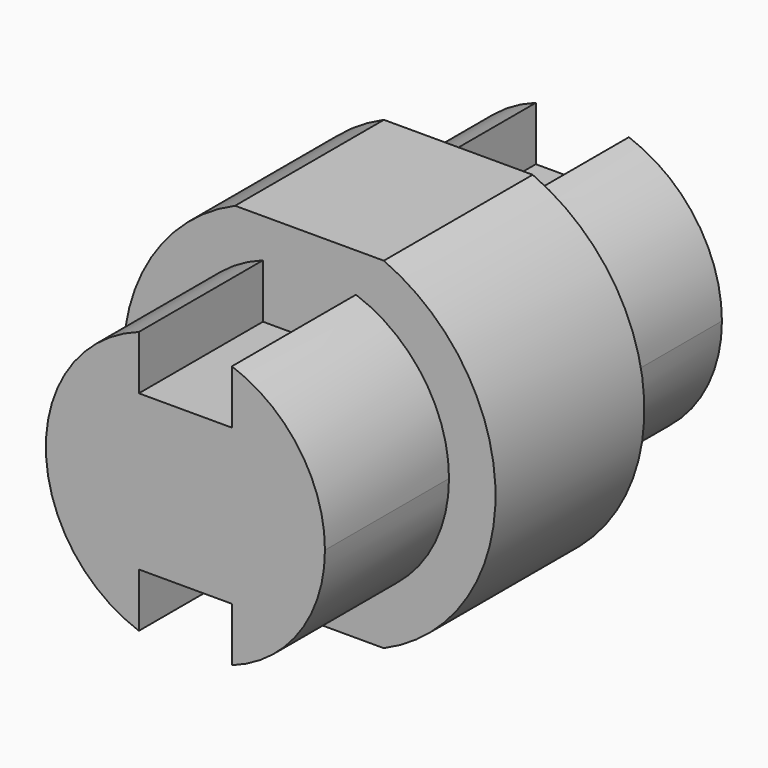
from build123d import *

# Parameters (mm, degrees)
F1_DEPTH = 15
F3_DEPTH = 25


# Not quite as in the source:
# - a pattern or mirror of a feature is missing from the dataset's text; its kind, count and spacing are read off the source's solid


with BuildPart() as f1:
    # F0 (on Front) → F1 (new body, symmetric)
    with BuildSketch(Plane.XZ):
        with BuildLine():
            ThreePointArc((11.9895788083, -27.5), (25.0966866762, -16.4364326384), (30, 0))
            ThreePointArc((30, 0), (25.0966866762, 16.4364326384), (11.9895788083, 27.5))
            Line((11.9895788083, 27.5), (-11.9895788083, 27.5))
            ThreePointArc((-11.9895788083, 27.5), (-30, 0), (-11.9895788083, -27.5))
            Line((-11.9895788083, -27.5), (11.9895788083, -27.5))
        make_face()
    extrude(amount=F1_DEPTH, both=True)

    # F2 (on face) → F3 (join)
    with BuildSketch(Plane.XZ.offset(15)):
        with BuildLine():
            ThreePointArc((7.5, -21.2132034356), (18.3711730709, -12.9903810568), (22.5, 0))
            ThreePointArc((22.5, 0), (18.3711730709, 12.9903810568), (7.5, 21.2132034356))
            Line((7.5, 21.2132034356), (7.5, 12.5))
            Line((7.5, 12.5), (-7.5, 12.5))
            Line((-7.5, 12.5), (-7.5, 21.2132034356))
            ThreePointArc((-7.5, 21.2132034356), (-22.5, 0), (-7.5, -21.2132034356))
            Line((-7.5, -21.2132034356), (-7.5, -12.5))
            Line((-7.5, -12.5), (7.5, -12.5))
            Line((7.5, -12.5), (7.5, -21.2132034356))
        make_face()
    f3 = extrude(amount=F3_DEPTH)

    # F3_copies: F3 across plane
    add(f3.mirror(Plane.ZX))


solid = f1.part
